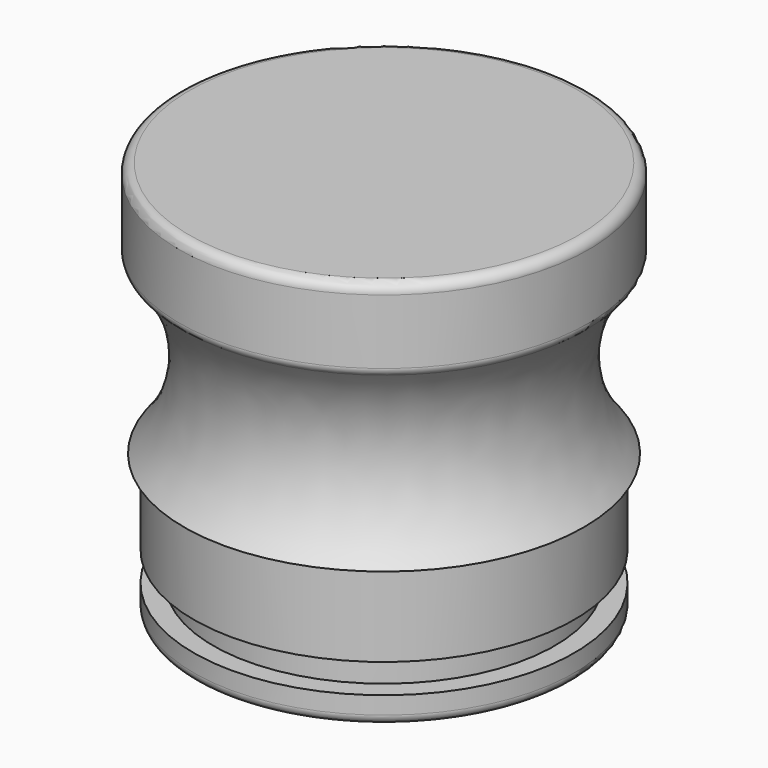
from build123d import *


# Not quite as in the source:
# - a fillet or chamfer that OpenCascade refuses, or shapes differently, is made with other operations: its cross-section is extruded or revolved along the edge and cut away or added


with BuildPart() as f1:
    # F0 (on Right) → F1 (revolve)
    with BuildSketch(Plane.YZ):
        with BuildLine():
            Line((7.5, 0), (7.5, -7.24))
            Line((7.5, -7.24), (9.75, -7.24))
            Line((9.75, -7.24), (9.75, -5.84))
            Line((9.75, -5.84), (8.75, -5.84))
            Line((8.75, -5.84), (8.75, -4.34))
            Line((8.75, -4.34), (9.75, -4.34))
            Line((9.75, -4.34), (9.75, 0))
            Line((9.75, 0), (10.25, 0))
            ThreePointArc((10.25, 0), (8.5974540278, 4.43), (10.25, 8.86))
            Line((10.25, 8.86), (10.5, 8.86))
            Line((10.5, 8.86), (10.5, 13.11))
            Line((10.5, 13.11), (0, 13.11))
            Line((0, 13.11), (0, 8.86))
            Line((0, 8.86), (0, 0))
            Line((0, 0), (7.5, 0))
        make_face()
    revolve(axis=Axis((0, 0, 4.43), (0, 0, 1)))

    # F2: fillet of radius 0.5 on 3 edges, made by hand

    # F2_s1 → F2_t2 (revolve, cut)
    with BuildSketch(Plane.YZ):
        with BuildLine():
            ThreePointArc((10.25, 8.86), (10.4330127019, 9.0430127019), (10.5, 9.2930127019))
            Line((10.5, 9.2930127019), (10.5, 8.86))
            Line((10.5, 8.86), (10.25, 8.86))
        make_face()
    revolve(axis=Axis((0, 0, 8.86), (0, 0, 1)), mode=Mode.SUBTRACT)

    # F2_s3 → F2_t4 (revolve, cut)
    with BuildSketch(Plane.YZ):
        with BuildLine():
            ThreePointArc((9.25, -7.24), (9.6035533906, -7.0935533906), (9.75, -6.74))
            Line((9.75, -6.74), (9.75, -7.24))
            Line((9.75, -7.24), (9.25, -7.24))
        make_face()
    revolve(axis=Axis((0, 0, -7.24), (0, 0, 1)), mode=Mode.SUBTRACT)

    # F2_s5 → F2_t6 (revolve, cut)
    with BuildSketch(Plane.YZ):
        with BuildLine():
            ThreePointArc((10.5, 12.61), (10.3535533906, 12.9635533906), (10, 13.11))
            Line((10, 13.11), (10.5, 13.11))
            Line((10.5, 13.11), (10.5, 12.61))
        make_face()
    revolve(axis=Axis((0, 0, 13.11), (0, 0, 1)), mode=Mode.SUBTRACT)


solid = f1.part
